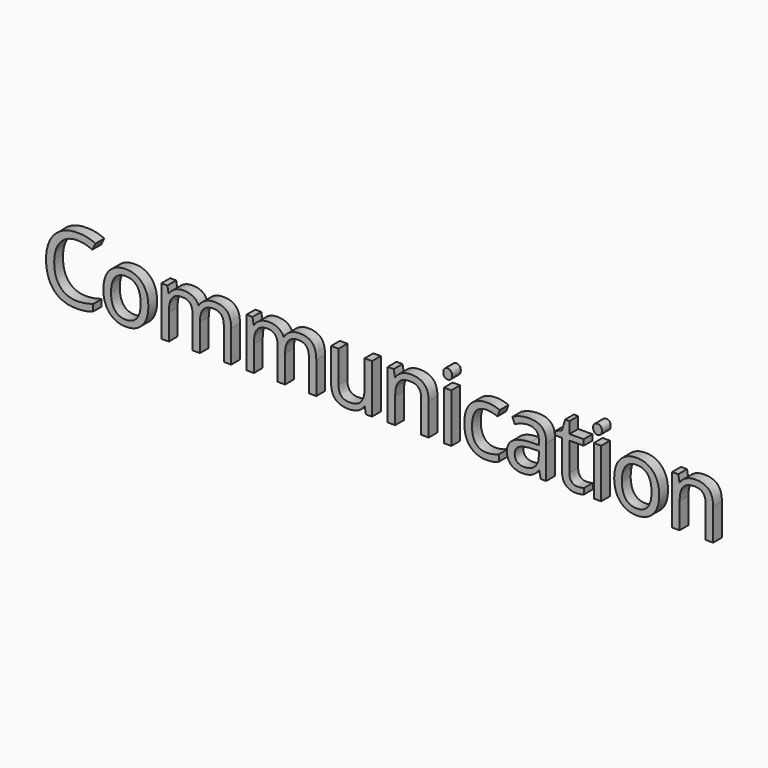
from build123d import *

# Parameters (mm, degrees)
F0_TEXT_SIZE = 211.5666452381
F1_DEPTH     = 25.4


# Not quite as in the source:
# - Text() gives the source's letters only with a copy of the font that has no kerning and outlines rounded to 1/6400 em; it was checked with that copy


with BuildPart() as f1:
    # F0 (on Front) → F1 (new body)
    with BuildSketch(Plane.XZ):
        with Locations((-76.3937160373, -76.2485340238)):
            Text('Communication', F0_TEXT_SIZE, font='Open Sans', text_align=(TextAlign.LEFT, TextAlign.BOTTOM))
    extrude(amount=F1_DEPTH)


solid = f1.part
